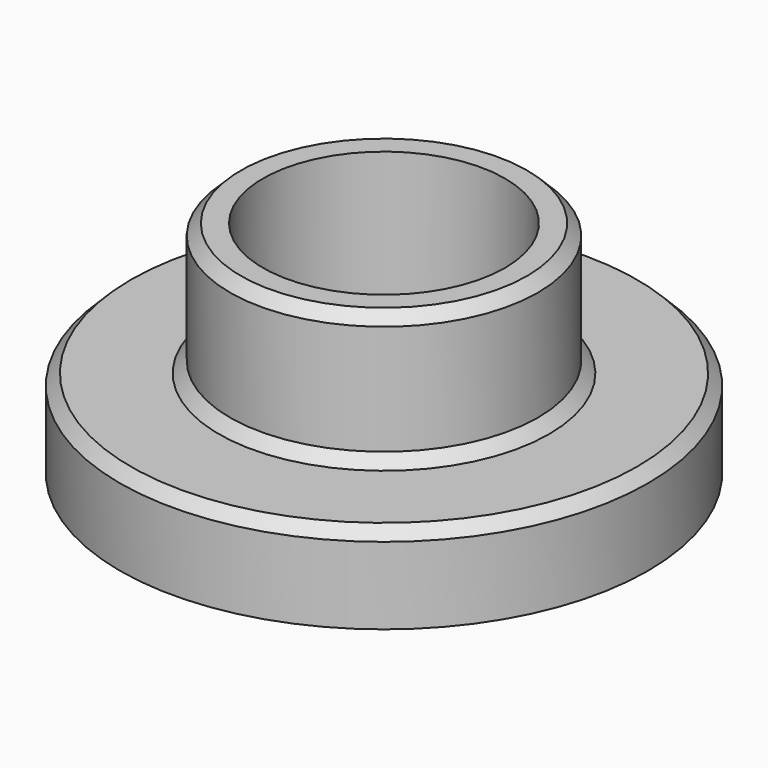
from build123d import *

# Parameters (mm, degrees)
F1_R     = 3.5
F1_R_2   = 2.75
F2_DEPTH = 5
F1_R_3   = 6
F3_DEPTH = 2
F4_SIZE  = 0.25


with BuildPart() as f2:
    # F1 (on Top) → F2 (new body)
    with BuildSketch(Plane.XY):
        Circle(F1_R)
        Circle(F1_R_2, mode=Mode.SUBTRACT)
    extrude(amount=F2_DEPTH)

    # F1 (on Top) → F3 (join)
    with BuildSketch(Plane.XY):
        Circle(F1_R_3)
        Circle(F1_R, mode=Mode.SUBTRACT)
    extrude(amount=F3_DEPTH)

    # F4
    f4_edges = [f2.edges().sort_by_distance(p)[0] for p in [
        (-3.5, 0, 5),
        (-3.5, 0, 2),
        (-6, 0, 2),
    ]]
    chamfer(f4_edges, length=F4_SIZE)


solid = f2.part
